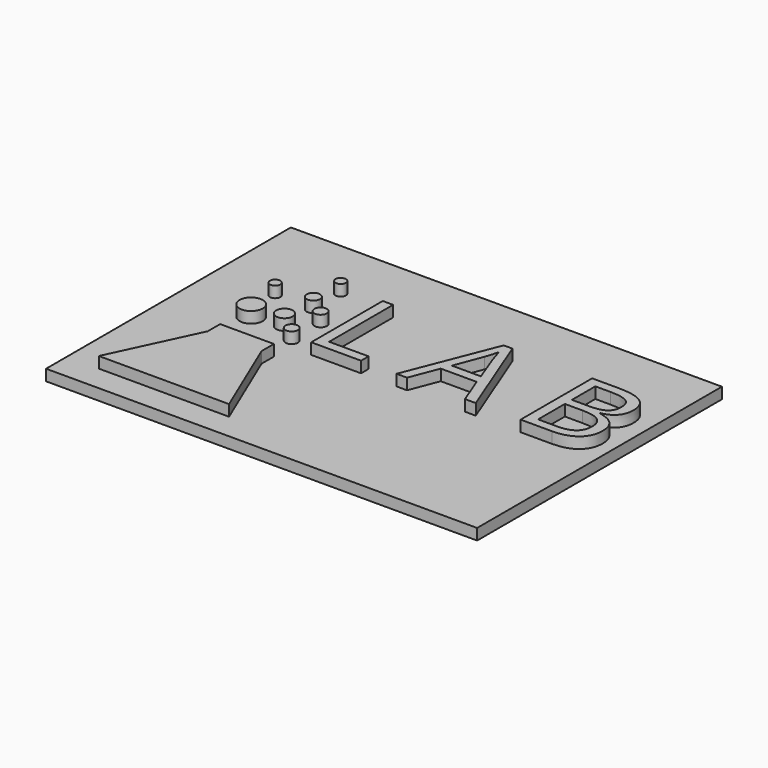
from build123d import *

# Parameters (mm, degrees)
F0_W         = 123.1150180101
F0_H         = 87.391000241
F1_DEPTH     = 3.175
F2_W         = 15.3524708003
F2_H         = 4.4285985641
F2_R         = 1.4761984348
F2_R_2       = 1.4761995524
F2_R_3       = 1.7714388669
F2_R_4       = 1.89045593
F2_R_5       = 3.3008802568
F2_R_6       = 2.3619178683
F4_DEPTH     = 6.35
F3_TEXT_SIZE = 35.7773336064
F5_DEPTH     = 3.175


# Not quite as in the source:
# - a length typed as a fraction of an inch, garbled in the dataset ("3 / 203.2 mm" for 3/8 in), is restored
# - Text() gives the source's letters only with a copy of the font that has no kerning and outlines rounded to 1/6400 em; it was checked with that copy


with BuildPart() as f1:
    # F0 (on Top) → F1 (new body)
    with BuildSketch(Plane.XY):
        with Locations((1.9928663969, 1.5500094742)):
            Rectangle(F0_W, F0_H)
    extrude(amount=F1_DEPTH)

    # F2 (on Top) → F4 (join)
    with BuildSketch(Plane.XY):
        Polygon((-38.8978496194, -10.2595854551), (-50.4122041166, -34.7644947469), (-13.211983256, -34.7644947469), (-23.5453788191, -10.2595854551), align=None)
        with Locations((-31.2216142192, -8.045286173)):
            Rectangle(F2_W, F2_H)
        with Locations((-41.8502502143, 17.4929611385)):
            Circle(F2_R)
        with Locations((-30.9263747185, 27.2358767688)):
            Circle(F2_R_2)
        with Locations((-25.316817686, 2.7309686411)):
            Circle(F2_R_3)
        with Locations((-30.9263747185, 17.4929611385)):
            Circle(F2_R_4)
        with Locations((-39.4883304834, 5.9786066413)):
            Circle(F2_R_5)
        with Locations((-25.316817686, 13.0643639714)):
            Circle(F2_R_3)
        with Locations((-30.9263747185, 7.1595665067)):
            Circle(F2_R_6)
    extrude(amount=F4_DEPTH)

    # F3 (on face) → F5 (join)
    with BuildSketch(Plane.XY.offset(3.175)):
        with Locations((-21.0683207855, 0)):
            Text('L A B', F3_TEXT_SIZE, font='Open Sans', text_align=(TextAlign.LEFT, TextAlign.BOTTOM))
    extrude(amount=F5_DEPTH)


solid = f1.part
